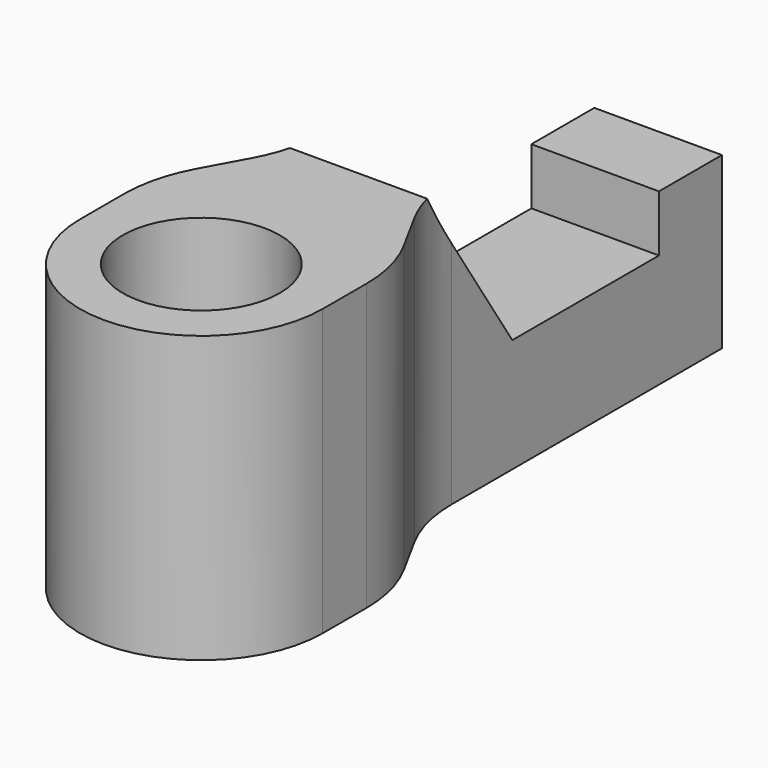
from build123d import *

# Parameters (mm, degrees)
F0_R     = 2.75
F1_DEPTH = 10
F3_DEPTH = 10
F4_F1_R  = 5
F4_F2_R  = 5
F4_F3_R  = 5
F4_F4_R  = 5


with BuildPart() as f1:
    # F0 (on Top) → F1 (new body)
    with BuildSketch(Plane.XY):
        with BuildLine():
            ThreePointArc((-4.25, 0), (0, 4.25), (4.25, 0))
            Line((4.25, 0), (4.25, 3.201806685))
            Line((4.25, 3.201806685), (2.2350018844, 6.8861790933))
            Line((2.2350018844, 6.8861790933), (2.2350018844, 10.8956433833))
            Line((2.2350018844, 10.8956433833), (2.2350018844, 20))
            Line((2.2350018844, 20), (-2.2350018844, 20))
            Line((-2.2350018844, 20), (-2.2350018844, 10.8956433833))
            Line((-2.2350018844, 10.8956433833), (-2.2350018844, 6.8861790933))
            Line((-2.2350018844, 6.8861790933), (-4.25, 3.201806685))
            Line((-4.25, 3.201806685), (-4.25, 0))
        make_face()
        with BuildLine():
            ThreePointArc((-4.25, 0), (0, -4.25), (4.25, 0))
            ThreePointArc((4.25, 0), (0, 4.25), (-4.25, 0))
        make_face()
        Circle(F0_R, mode=Mode.SUBTRACT)
    extrude(amount=F1_DEPTH)

    # F2 (on face) → F3 (cut)
    with BuildSketch(Plane(origin=(-2.2350018844, 0, 0), x_dir=(0, -1, 0), z_dir=(-1, 0, 0))):
        Polygon((-10.8234519139, 3.9840904064), (-6.8861790933, 10), (-20, 10), (-20, 5.9617315419), (-17.2440130264, 5.9617315419), (-17.2440130264, 3.9840904064), align=None)
    extrude(amount=-F3_DEPTH, mode=Mode.SUBTRACT)

    # F4: fillet of radius 5 on 6 edges, made by hand

    # F4_f1
    f4_f1_edges = [f1.edges().sort_by_distance(p)[0] for p in [
        (-4.25, 3.201806685, 5),
    ]]
    fillet(f4_f1_edges, radius=F4_F1_R)

    # F4_f2
    f4_f2_edges = [f1.edges().sort_by_distance(p)[0] for p in [
        (-2.2350018844, 6.8861790933, 5),
    ]]
    fillet(f4_f2_edges, radius=F4_F2_R)

    # F4_f3
    f4_f3_edges = [f1.edges().sort_by_distance(p)[0] for p in [
        (4.25, 3.201806685, 5),
    ]]
    fillet(f4_f3_edges, radius=F4_F3_R)

    # F4_f4
    f4_f4_edges = [f1.edges().sort_by_distance(p)[0] for p in [
        (2.2350018844, 6.8861790933, 5),
    ]]
    fillet(f4_f4_edges, radius=F4_F4_R)


solid = f1.part
